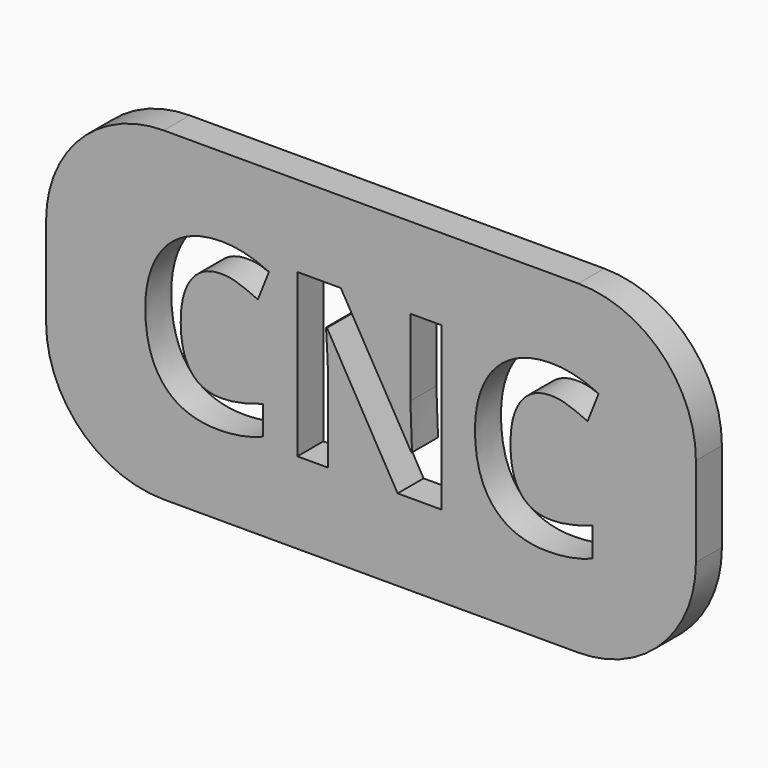
from build123d import *

# Parameters (mm, degrees)
F0_W         = 101.6
F0_H         = 50.8
F1_DEPTH     = 5.08
F2_R         = 18.3963073453
F3_TEXT_SIZE = 35.5456399524
F4_DEPTH     = 5.08


# Not quite as in the source:
# - Text() gives the source's letters only with a copy of the font that has no kerning and outlines rounded to 1/6400 em; it was checked with that copy


with BuildPart() as f1:
    # F0 (on Front) → F1 (new body)
    with BuildSketch(Plane.XZ):
        Rectangle(F0_W, F0_H)
    extrude(amount=F1_DEPTH)

    # F2
    f2_edges = [f1.edges().sort_by_distance(p)[0] for p in [
        (-50.8, -2.54, 25.4),
        (50.8, -2.54, 25.4),
        (50.8, -2.54, -25.4),
        (-50.8, -2.54, -25.4),
    ]]
    fillet(f2_edges, radius=F2_R)

    # F3 (on face) → F4 (cut, through all)
    with BuildSketch(Plane.XZ.offset(5.08)):
        with Locations((-37.3552329838, -12.6671735197)):
            Text('CNC', F3_TEXT_SIZE, font='Open Sans', font_style=FontStyle.BOLD, text_align=(TextAlign.LEFT, TextAlign.BOTTOM))
    extrude(amount=-F4_DEPTH, mode=Mode.SUBTRACT)


solid = f1.part
